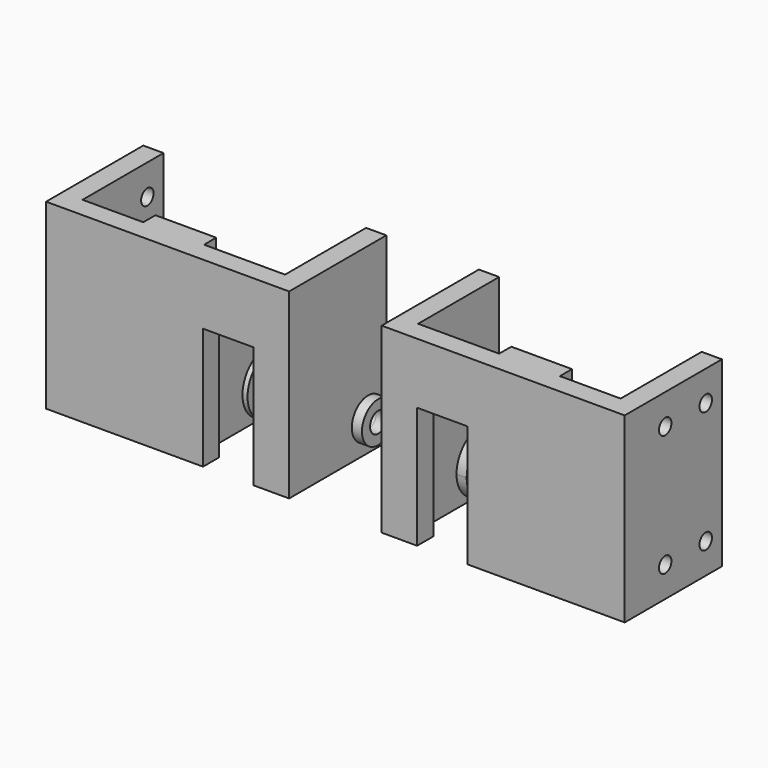
from build123d import *
from build123d import SkipClean  # not in build123d's __all__

# Parameters (mm, degrees)
F1_DEPTH  = 3.175
F2_W      = 3.175
F2_H      = 28.575
F3_DEPTH  = 15.875
F4_W      = 3.175
F4_H      = 28.575
F5_DEPTH  = 15.875
F6_W      = 9.525
F6_H      = 28.575
F7_DEPTH  = 2.38125
F8_W      = 2.38125
F8_H      = 28.575
F9_DEPTH  = 15.08125
F11_DEPTH = 2.38125
F12_R     = 4.7625
F13_R     = 4.7625
F14_DEPTH = 0.79375
F15_R     = 3.175
F16_DEPTH = 1.5875
F17_R     = 1.5875
F18_DEPTH = 25.4
F19_R     = 1.5875
F20_DEPTH = 1.5875
F21_R     = 3.175
F21_R_2   = 1.5875
F22_DEPTH = 1.5875
F23_R     = 1.2192
F24_DEPTH = 4.7625
F26_DEPTH = 1.190625


# Not quite as in the source:
# - after a boolean that leaves OpenCascade's solid faulty, fix() repairs it


with BuildPart() as f1:
    # F0 (on Front) → F1 (new body)
    with BuildSketch(Plane.XZ):
        Polygon((-12.810901, 0), (-7.254651, 0), (-7.254651, 28.575), (-45.354651, 28.575), (-45.354651, 0), (-20.748401, 0), (-20.748401, 19.05), (-12.810901, 19.05), align=None)
    extrude(amount=F1_DEPTH)

    # F2 (on face) → F3 (join)
    with BuildSketch(Plane(origin=(0, 0, 0), x_dir=(-1, 0, 0), z_dir=(0, 1, 0))):
        with Locations((43.767151, 14.2875)):
            Rectangle(F2_W, F2_H)
    extrude(amount=F3_DEPTH)

    # F4 (on face) → F5 (join)
    with BuildSketch(Plane(origin=(0, 0, 0), x_dir=(-1, 0, 0), z_dir=(0, 1, 0))):
        with Locations((8.842151, 14.2875)):
            Rectangle(F4_W, F4_H)
    extrude(amount=F5_DEPTH)

    # F6 (on face) → F7 (join)
    with BuildSketch(Plane(origin=(0, 0, 0), x_dir=(-1, 0, 0), z_dir=(0, 1, 0))):
        with Locations((27.892151, 14.2875)):
            Rectangle(F6_W, F6_H)
    extrude(amount=F7_DEPTH)

    # F8 (on face) → F9 (join)
    with BuildSketch(Plane(origin=(0, 2.38125, 0), x_dir=(-1, 0, 0), z_dir=(0, 1, 0))):
        with Locations((24.320276, 14.2875)):
            Rectangle(F8_W, F8_H)
    extrude(amount=F9_DEPTH)

    # F10 (on face) → F11 (cut)
    with BuildSketch(Plane.YZ.offset(-23.129651)):
        with BuildLine():
            ThreePointArc((15.657919, 8.130096), (16.690299, 6.58503), (17.052823, 4.7625))
            ThreePointArc((17.052823, 4.7625), (15.657919, 1.394904), (12.290323, 0))
            Line((12.290323, 0), (17.4625, 0))
            Line((17.4625, 0), (17.4625, 28.575))
            Line((17.4625, 28.575), (2.38125, 28.575))
            Line((2.38125, 28.575), (2.38125, 21.406765))
            Line((2.38125, 21.406765), (15.657919, 8.130096))
        make_face()
    extrude(amount=-F11_DEPTH, mode=Mode.SUBTRACT)

    # F12
    f12_edges = [f1.edges().sort_by_distance(p)[0] for p in [
        (-24.320276, 2.38125, 21.406765),
    ]]
    fillet(f12_edges, radius=F12_R)

    # F13 (on face) → F14 (join)
    with BuildSketch(Plane.YZ.offset(-23.129651)):
        with Locations((12.290323, 4.7625)):
            Circle(F13_R)
    extrude(amount=F14_DEPTH)

    # F15 (on face) → F16 (join)
    with BuildSketch(Plane(origin=(-25.510901, 0, 0), x_dir=(0, -1, 0), z_dir=(-1, 0, 0))):
        with Locations((-12.290323, 4.7625)):
            Circle(F15_R)
    extrude(amount=F16_DEPTH)

    # F17 (on face) → F18 (cut)
    with BuildSketch(Plane(origin=(-27.098401, 0, 0), x_dir=(0, -1, 0), z_dir=(-1, 0, 0))):
        with Locations((-12.290323, 4.7625)):
            Circle(F17_R)
    extrude(amount=-F18_DEPTH, mode=Mode.SUBTRACT)

    # F19 (on face) → F20 (join)
    with BuildSketch(Plane(origin=(-10.429651, 0, 0), x_dir=(0, -1, 0), z_dir=(-1, 0, 0))):
        with BuildLine():
            ThreePointArc((-12.290323, 0), (-8.922727, 1.394904), (-7.527823, 4.7625))
            ThreePointArc((-7.527823, 4.7625), (-10.615602, 9.220831), (-15.875, 7.898021))
            Line((-15.875, 7.898021), (-15.875, 1.626979))
            ThreePointArc((-15.875, 1.626979), (-14.258632, 0.425777), (-12.290323, 0))
        make_face()
        with Locations((-12.290323, 4.7625)):
            Circle(F19_R, mode=Mode.SUBTRACT)
        with BuildLine():
            Line((-15.875, 1.626979), (-15.875, 7.898021))
            ThreePointArc((-15.875, 7.898021), (-17.052823, 4.7625), (-15.875, 1.626979))
        make_face()
    extrude(amount=F20_DEPTH)

    # F21 (on face) → F22 (join)
    with BuildSketch(Plane.YZ.offset(-7.254651)):
        with Locations((12.290323, 4.7625)):
            Circle(F21_R)
        with Locations((12.290323, 4.7625)):
            Circle(F21_R_2, mode=Mode.SUBTRACT)
    with SkipClean():  # cleaning this boolean's faces spoils the solid; the shape is the same uncleaned
        extrude(amount=F22_DEPTH)

    # F23 (on face) → F24 (cut)
    with BuildSketch(Plane(origin=(-45.354651, 0, 0), x_dir=(0, -1, 0), z_dir=(-1, 0, 0))):
        with Locations((-12.7, 23.8125)):
            Circle(F23_R)
        with Locations((-4.7625, 23.8125)):
            Circle(F23_R)
        with Locations((-12.7, 4.7625)):
            Circle(F23_R)
        with Locations((-4.7625, 4.7625)):
            Circle(F23_R)
    extrude(amount=-F24_DEPTH, mode=Mode.SUBTRACT)

    add(f1.part.fix(), mode=Mode.REPLACE)

    # F25 (on face) → F26 (join)
    with BuildSketch(Plane(origin=(0, 2.38125, 0), x_dir=(-1, 0, 0), z_dir=(0, 1, 0))):
        Polygon((29.992783, 22.846448), (31.260251, 24.170734), (30.747119, 25.930536), (28.96652, 26.366052), (27.699052, 25.041766), (28.212184, 23.281964), align=None)
        Polygon((28.980526, 2.204924), (30.757607, 2.654582), (31.256732, 4.418408), (29.978777, 5.732576), (28.201696, 5.282918), (27.702571, 3.519092), align=None)
    extrude(amount=F26_DEPTH)


with BuildPart() as f27_1:
    # F27: instance of F1
    add(f1.part.mirror(Plane.YZ), clean=False)


solid = Compound([f1.part, f27_1.part])
